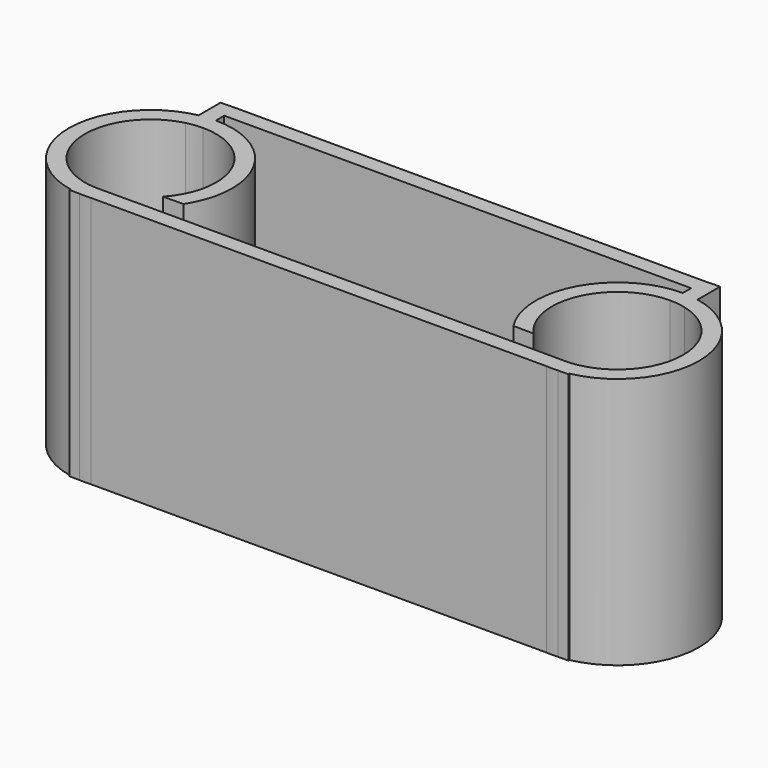
from build123d import *

# Parameters (mm, degrees)
F0_W     = 88.9
F0_H     = 3
F1_DEPTH = 24
F3_R     = 3.81
F5_DEPTH = 3.048
F4_R     = 12.7
F6_DEPTH = 2.794


with BuildPart() as f1:
    # F0 (on Top) → F1 (new body, symmetric)
    with BuildSketch(Plane.XY):
        with Locations((0, 16.5)):
            Rectangle(F0_W, F0_H)
        with BuildLine():
            Line((-44.45, 13.008), (-44.45, 15))
            Line((-44.45, 15), (-44.45, 18))
            Line((-44.45, 18), (-47.498, 17.941171))
            Line((-47.498, 17.941171), (-47.498, 12.706311))
            ThreePointArc((-47.498, 12.706311), (-45.981447, 12.932394), (-44.45, 13.008))
        make_face()
        with BuildLine():
            Line((44.45, 18), (44.45, 15))
            Line((44.45, 15), (44.45, 13.008))
            ThreePointArc((44.45, 13.008), (45.981447, 12.932394), (47.498, 12.706311))
            Line((47.498, 12.706311), (47.498, 18.075556))
            Line((47.498, 18.075556), (44.45, 18))
        make_face()
        with BuildLine():
            Line((-44.45, 9.96), (-44.45, 13.008))
            ThreePointArc((-44.45, 13.008), (-45.981447, 12.932394), (-47.498, 12.706311))
            Line((-47.498, 12.706311), (-47.498, 9.582693))
            ThreePointArc((-47.498, 9.582693), (-45.985632, 9.865315), (-44.45, 9.96))
        make_face()
        with BuildLine():
            ThreePointArc((47.498, 12.706311), (45.981447, 12.932394), (44.45, 13.008))
            Line((44.45, 13.008), (44.45, 9.96))
            ThreePointArc((44.45, 9.96), (45.985632, 9.865315), (47.498, 9.582693))
            Line((47.498, 9.582693), (47.498, 12.706311))
        make_face()
        with BuildLine():
            Line((-47.498, 9.582693), (-47.498, 12.706311))
            ThreePointArc((-47.498, 12.706311), (-59.998, -2.54), (-47.498, -17.786311))
            Line((-47.498, -17.786311), (-47.498, -14.662693))
            ThreePointArc((-47.498, -14.662693), (-56.95, -2.54), (-47.498, 9.582693))
        make_face()
        with BuildLine():
            ThreePointArc((47.498, -17.786311), (59.998, -2.54), (47.498, 12.706311))
            Line((47.498, 12.706311), (47.498, 9.582693))
            ThreePointArc((47.498, 9.582693), (56.95, -2.54), (47.498, -14.662693))
            Line((47.498, -14.662693), (47.498, -17.786311))
        make_face()
        with BuildLine():
            ThreePointArc((-45.564556, -18.048), (-46.535387, -17.947513), (-47.498, -17.786311))
            Line((-47.498, -17.786311), (-47.498, -18.048))
            Line((-47.498, -18.048), (-45.564556, -18.048))
        make_face()
        with BuildLine():
            Line((-47.498, -14.662693), (-47.498, -17.786311))
            ThreePointArc((-47.498, -17.786311), (-46.535387, -17.947513), (-45.564556, -18.048))
            Line((-45.564556, -18.048), (-43.335444, -18.048))
            ThreePointArc((-43.335444, -18.048), (-39.024324, -17.110599), (-35.15007, -15))
            Line((-35.15007, -15), (-44.428119, -15.039981))
            ThreePointArc((-44.428119, -15.039981), (-45.974774, -14.946654), (-47.498, -14.662693))
        make_face()
        with BuildLine():
            ThreePointArc((45.564558, -18.048), (46.535388, -17.947513), (47.498, -17.786311))
            Line((47.498, -17.786311), (47.498, -14.662693))
            ThreePointArc((47.498, -14.662693), (46.043463, -14.938019), (44.566576, -15.039456))
            ThreePointArc((44.566576, -15.039456), (44.397624, -15.03989), (44.228681, -15.038041))
            Line((44.228681, -15.038041), (35.15007, -15))
            ThreePointArc((35.15007, -15), (39.024323, -17.110598), (43.335442, -18.048))
            Line((43.335442, -18.048), (45.564558, -18.048))
        make_face()
        with BuildLine():
            Line((47.498, -18.048), (47.498, -17.786311))
            ThreePointArc((47.498, -17.786311), (46.535388, -17.947513), (45.564558, -18.048))
            Line((45.564558, -18.048), (47.498, -18.048))
        make_face()
        with BuildLine():
            Line((-43.335444, -18.048), (-45.564556, -18.048))
            ThreePointArc((-45.564556, -18.048), (-44.45, -18.088), (-43.335444, -18.048))
        make_face()
        with BuildLine():
            ThreePointArc((43.335442, -18.048), (44.45, -18.088), (45.564558, -18.048))
            Line((45.564558, -18.048), (43.335442, -18.048))
        make_face()
        with BuildLine():
            Line((35.15007, -15), (-35.15007, -15))
            ThreePointArc((-35.15007, -15), (-39.024324, -17.110599), (-43.335444, -18.048))
            Line((-43.335444, -18.048), (43.335442, -18.048))
            ThreePointArc((43.335442, -18.048), (39.024323, -17.110598), (35.15007, -15))
        make_face()
        with BuildLine():
            Line((44.45, 9.96), (44.45, 13.008))
            ThreePointArc((44.45, 13.008), (30.788441, 4.88308), (31.405127, -11))
            Line((31.405127, -11), (35.284344, -11.039456))
            ThreePointArc((35.284344, -11.039456), (32.993709, 2.46034), (44.45, 9.96))
        make_face()
        with BuildLine():
            ThreePointArc((-31.405127, -11), (-30.788441, 4.88308), (-44.45, 13.008))
            Line((-44.45, 13.008), (-44.45, 9.96))
            ThreePointArc((-44.45, 9.96), (-32.993566, 2.460012), (-35.284831, -11.039981))
            Line((-35.284831, -11.039981), (-31.405127, -11))
        make_face()
    extrude(amount=F1_DEPTH, both=True)

    # F3 (on offset) → F5 (cut)
    with BuildSketch(Plane.XZ.offset(-18.047995)):
        Circle(F3_R)
    extrude(amount=F5_DEPTH, mode=Mode.SUBTRACT)

    # F4 (on offset) → F6 (cut)
    with BuildSketch(Plane.XZ.offset(-18.047995)):
        Circle(F4_R)
    extrude(amount=F6_DEPTH, mode=Mode.SUBTRACT)


solid = f1.part
